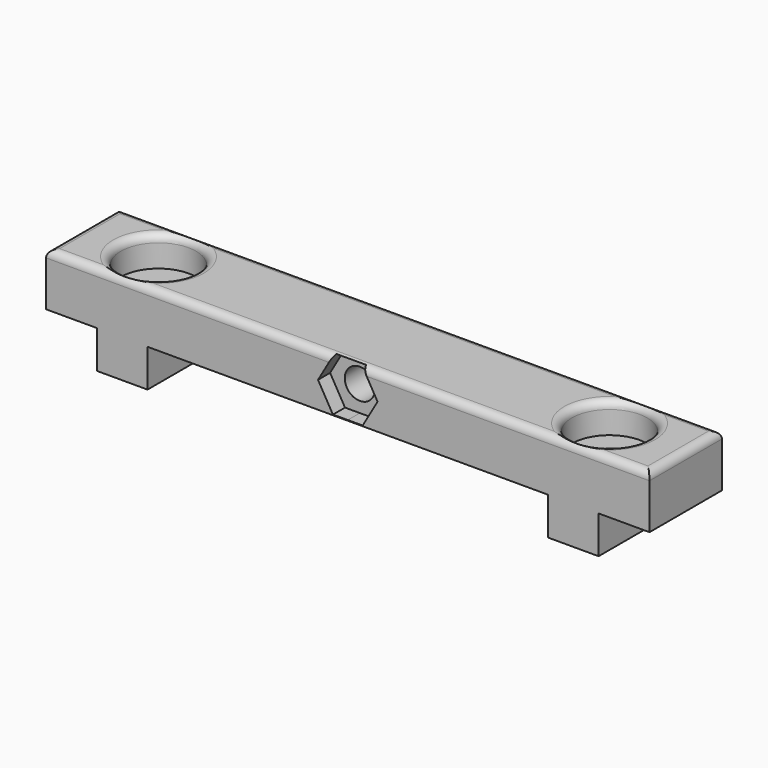
from build123d import *

# Parameters (mm, degrees)
F0_W           = 3.35
F0_H           = 5
F1_DEPTH       = 12
F3_D           = 4
F3_DEPTH       = 25
F3_CBORE_D     = 10
F3_CBORE_DEPTH = 4
F3_TIP         = 1.2017212381
F5_D           = 4
F5_DEPTH       = 25
F5_TIP         = 1.2017212381
F6_DEPTH       = 2
F7_T1_DEPTH    = 17
F7_T3_DEPTH    = 85


# Not quite as in the source:
# - a fillet or chamfer that OpenCascade refuses, or shapes differently, is made with other operations: its cross-section is extruded or revolved along the edge and cut away or added


with BuildPart() as f1:
    # F0 (on Front) → F1 (new body)
    with BuildSketch(Plane.XZ):
        with Locations((8.425, 2.5)):
            Rectangle(F0_W, F0_H)
        with Locations((11.775, 2.5)):
            Rectangle(F0_W, F0_H)
        Polygon((0, 5), (6.75, 5), (10.1, 5), (10.1, 12), (0, 12), align=None)
        Polygon((10.1, 12), (10.1, 5), (13.45, 5), (66.55, 5), (69.9, 5), (69.9, 12), align=None)
        with Locations((68.225, 2.5)):
            Rectangle(F0_W, F0_H)
        Polygon((80, 12), (69.9, 12), (69.9, 5), (73.25, 5), (80, 5), align=None)
        with Locations((71.575, 2.5)):
            Rectangle(F0_W, F0_H)
    extrude(amount=F1_DEPTH)

    # F3
    with Locations(Plane.XY.offset(12)):
        with Locations((10.1, -6), (69.9, -6)):
            CounterBoreHole(F3_D / 2, F3_CBORE_D / 2, F3_CBORE_DEPTH, depth=F3_DEPTH)
            with Locations((0, 0, -(F3_DEPTH + F3_TIP / 2))):  # 118° drill point
                Cone(0, F3_D / 2, F3_TIP, mode=Mode.SUBTRACT)

    # F5
    with Locations(Plane.XZ.offset(12)):
        with Locations((40, 8.5)):
            Hole(F5_D / 2, depth=F5_DEPTH)
            with Locations((0, 0, -(F5_DEPTH + F5_TIP / 2))):  # 118° drill point
                Cone(0, F5_D / 2, F5_TIP, mode=Mode.SUBTRACT)

    # F4 (on face) → F6 (cut)
    with BuildSketch(Plane.XZ.offset(12)):
        with BuildLine():
            Line((38.0252040749, 11.9131824428), (36.0587919372, 8.5))
            Line((36.0587919372, 8.5), (38.5835167795, 8.5))
            ThreePointArc((38.5835167795, 8.5), (38.9983951094, 9.5016048906), (40, 9.9164832205))
            Line((40, 9.9164832205), (40, 11.9150014487))
            Line((40, 11.9150014487), (38.0252040749, 11.9131824428))
        make_face()
        with BuildLine():
            Line((38.5835167795, 8.5), (36.0587919372, 8.5))
            Line((36.0587919372, 8.5), (36.0566993343, 8.496367783))
            Line((36.0566993343, 8.496367783), (38.0314952594, 5.0831853402))
            Line((38.0314952594, 5.0831853402), (40, 5.0849985513))
            Line((40, 5.0849985513), (40, 7.0835167795))
            ThreePointArc((40, 7.0835167795), (38.9983951094, 7.4983951094), (38.5835167795, 8.5))
        make_face()
        with BuildLine():
            Line((40, 11.9150014487), (40, 9.9164832205))
            ThreePointArc((40, 9.9164832205), (41.0016048906, 9.5016048906), (41.4164832205, 8.5))
            Line((41.4164832205, 8.5), (43.9412080628, 8.5))
            Line((43.9412080628, 8.5), (43.9433006657, 8.503632217))
            Line((43.9433006657, 8.503632217), (41.9685047406, 11.9168146598))
            Line((41.9685047406, 11.9168146598), (40, 11.9150014487))
        make_face()
        with BuildLine():
            ThreePointArc((41.4164832205, 8.5), (41.0016048906, 7.4983951094), (40, 7.0835167795))
            Line((40, 7.0835167795), (40, 5.0849985513))
            Line((40, 5.0849985513), (41.9747959251, 5.0868175572))
            Line((41.9747959251, 5.0868175572), (43.9412080628, 8.5))
            Line((43.9412080628, 8.5), (41.4164832205, 8.5))
        make_face()
    extrude(amount=-F6_DEPTH, mode=Mode.SUBTRACT)

    # F7: fillet of radius 1 on 6 edges, made by hand

    # F7_s2 → F7_t1 (cut)
    with BuildSketch(Plane.XZ.offset(-2.5)):
        with BuildLine():
            ThreePointArc((79, 12), (79.7071067812, 11.7071067812), (80, 11))
            Line((80, 11), (80, 12))
            Line((80, 12), (79, 12))
        make_face()
        with BuildLine():
            ThreePointArc((0, 11), (0.2928932188, 11.7071067812), (1, 12))
            Line((1, 12), (0, 12))
            Line((0, 12), (0, 11))
        make_face()
    extrude(amount=F7_T1_DEPTH, mode=Mode.SUBTRACT)

    # F7_s4 → F7_t3 (cut)
    with BuildSketch(Plane.YZ.offset(-2.5)):
        with BuildLine():
            ThreePointArc((0, 11), (-0.2928932188, 11.7071067812), (-1, 12))
            Line((-1, 12), (0, 12))
            Line((0, 12), (0, 11))
        make_face()
        with BuildLine():
            ThreePointArc((-12, 11), (-11.7071067812, 11.7071067812), (-11, 12))
            Line((-11, 12), (-12, 12))
            Line((-12, 12), (-12, 11))
        make_face()
    extrude(amount=F7_T3_DEPTH, mode=Mode.SUBTRACT)

    # F7_s5 → F7_t6 (revolve, cut)
    with BuildSketch(Plane.XZ.offset(6)):
        with BuildLine():
            ThreePointArc((75.9, 12), (75.1928932188, 11.7071067812), (74.9, 11))
            Line((74.9, 11), (74.9, 12))
            Line((74.9, 12), (75.9, 12))
        make_face()
    revolve(axis=Axis((69.9, -6, 12), (0, 0, 1)), mode=Mode.SUBTRACT)

    # F7_s7 → F7_t8 (revolve, cut)
    with BuildSketch(Plane.XZ.offset(6)):
        with BuildLine():
            ThreePointArc((16.1, 12), (15.3928932188, 11.7071067812), (15.1, 11))
            Line((15.1, 11), (15.1, 12))
            Line((15.1, 12), (16.1, 12))
        make_face()
    revolve(axis=Axis((10.1, -6, 12), (0, 0, 1)), mode=Mode.SUBTRACT)


solid = f1.part
